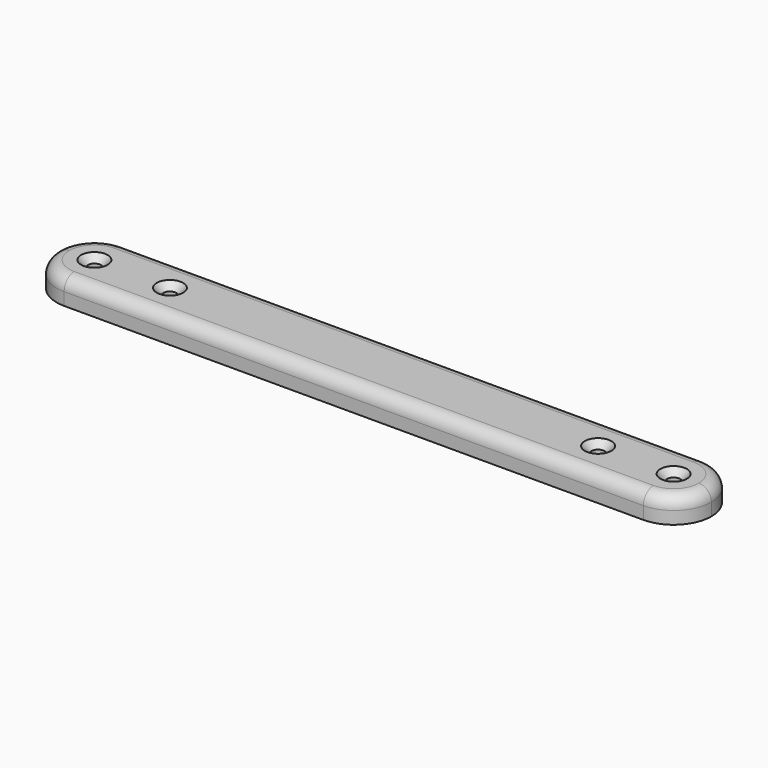
from build123d import *

# Parameters (mm, degrees)
F0_R     = 1.67
F1_DEPTH = 6.35
F2_R     = 3.175
F3_SIZE  = 1.675


with BuildPart() as f1:
    # F0 (on Top) → F1 (new body)
    with BuildSketch(Plane.XY):
        with BuildLine():
            Line((73.025, 9.525), (63.5, 9.525))
            Line((63.5, 9.525), (-63.5, 9.525))
            Line((-63.5, 9.525), (-73.025, 9.525))
            ThreePointArc((-73.025, 9.525), (-79.7601920908, 6.7351920908), (-82.55, 0))
            ThreePointArc((-82.55, 0), (-79.7601920908, -6.7351920908), (-73.025, -9.525))
            Line((-73.025, -9.525), (-63.5, -9.525))
            Line((-63.5, -9.525), (63.5, -9.525))
            Line((63.5, -9.525), (73.025, -9.525))
            ThreePointArc((73.025, -9.525), (79.7601920908, -6.7351920908), (82.55, 0))
            ThreePointArc((82.55, 0), (79.7601920908, 6.7351920908), (73.025, 9.525))
        make_face()
        with Locations((-73.025, 0)):
            Circle(F0_R, mode=Mode.SUBTRACT)
        with Locations((-53.975, 0)):
            Circle(F0_R, mode=Mode.SUBTRACT)
        with Locations((53.975, 0)):
            Circle(F0_R, mode=Mode.SUBTRACT)
        with Locations((73.025, 0)):
            Circle(F0_R, mode=Mode.SUBTRACT)
    extrude(amount=F1_DEPTH)

    # F2
    f2_edges = [f1.edges().sort_by_distance(p)[0] for p in [
        (-82.55, 0, 6.35),
        (82.55, 0, 6.35),
        (0, 9.525, 6.35),
        (0, -9.525, 6.35),
    ]]
    fillet(f2_edges, radius=F2_R)

    # F3
    f3_edges = [f1.edges().sort_by_distance(p)[0] for p in [
        (-74.695, 0, 6.35),
        (-55.645, 0, 6.35),
        (52.305, 0, 6.35),
        (71.355, 0, 6.35),
    ]]
    chamfer(f3_edges, length=F3_SIZE)


solid = f1.part
